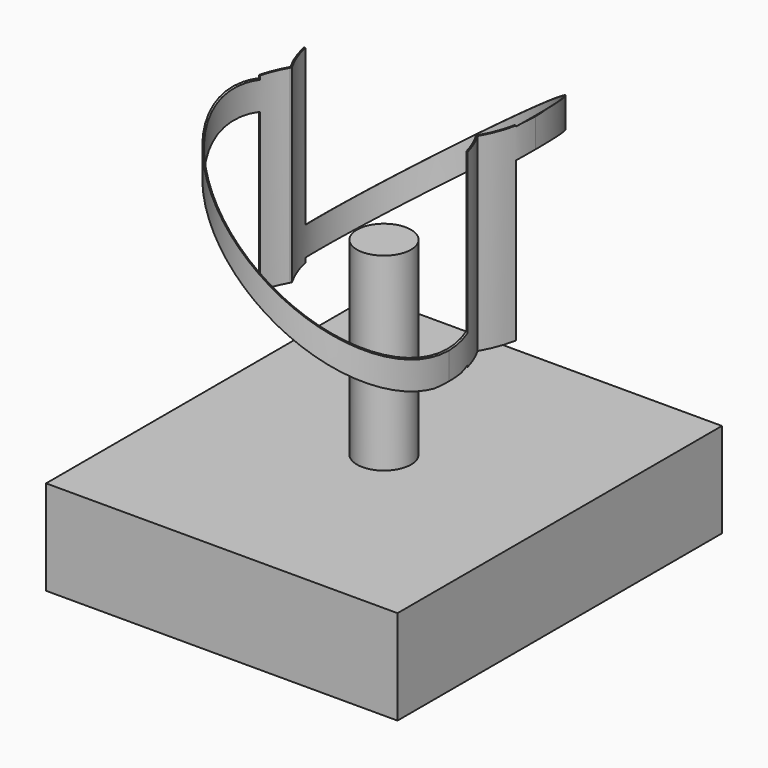
from build123d import *

# Parameters (mm, degrees)
F1_DEPTH = 35
F2_R     = 10
F3_DEPTH = 45
F5_DEPTH = 70
F7_DEPTH = 63
F9_DEPTH = 65.4


with BuildPart() as f1:
    # F0 (on Top) → F1 (new body)
    with BuildSketch(Plane.XY):
        Polygon((-147.9383396478, 75), (-147.9383396478, 0), (-147.9383396478, -75), (-17.9383396478, -75), (-17.9383396478, 0), (-17.9383396478, 75), align=None)
    extrude(amount=F1_DEPTH)

    # F2 (on face) → F3 (join)
    with BuildSketch(Plane.XY.offset(35)):
        with Locations((-82.9383396478, 0)):
            Circle(F2_R)
    extrude(amount=F3_DEPTH)

    # F2 (on face) → F5, piece 2 (join)
    with BuildSketch(Plane.XY.offset(35)):
        with Locations((-82.9383396478, 0)):
            Circle(F2_R)
    extrude(amount=F5_DEPTH)


with BuildPart() as f5:
    # F4 (on face) → F5 (new body)
    with BuildSketch(Plane.XY.offset(80)):
        with BuildLine():
            ThreePointArc((-48.5889857203, 0.496875), (-48.7315391647, 0.2479165476), (-48.8758969873, 0))
            ThreePointArc((-48.8758969873, 0), (-48.7315391647, -0.2479165476), (-48.5889857203, -0.496875))
            ThreePointArc((-48.5889857203, -0.496875), (-48.4422599851, -0.2489626377), (-48.2973234964, 0))
            ThreePointArc((-48.2973234964, 0), (-48.4422599851, 0.2489626377), (-48.5889857203, 0.496875))
        make_face()
        with BuildLine():
            ThreePointArc((-117.2876935753, -0.496875), (-117.1451401309, -0.2479165476), (-117.0007823083, 0))
            ThreePointArc((-117.0007823083, 0), (-117.1451401309, 0.2479165476), (-117.2876935753, 0.496875))
            ThreePointArc((-117.2876935753, 0.496875), (-117.4344193105, 0.2489626377), (-117.5793557992, 0))
            ThreePointArc((-117.5793557992, 0), (-117.4344193105, -0.2489626377), (-117.2876935753, -0.496875))
        make_face()
        with BuildLine():
            ThreePointArc((-43.4383396478, 20), (-44.7477028363, 9.9141058933), (-48.5889857203, 0.496875))
            ThreePointArc((-48.5889857203, 0.496875), (-48.4422599851, 0.2489626377), (-48.2973234964, 0))
            ThreePointArc((-48.2973234964, 0), (-44.3013065963, 9.6472381959), (-42.9383396478, 20))
            ThreePointArc((-42.9383396478, 20), (-93.2911014519, 58.6370330516), (-117.5793557992, 0))
            ThreePointArc((-117.5793557992, 0), (-117.4344193105, 0.2489626377), (-117.2876935753, 0.496875))
            ThreePointArc((-117.2876935753, 0.496875), (-93.0242337546, 58.1906368115), (-43.4383396478, 20))
        make_face()
        with BuildLine():
            ThreePointArc((-48.2973234964, 0), (-48.4422599851, -0.2489626377), (-48.5889857203, -0.496875))
            ThreePointArc((-48.5889857203, -0.496875), (-44.7477028363, -9.9141058933), (-43.4383396478, -20))
            ThreePointArc((-43.4383396478, -20), (-93.0242337546, -58.1906368115), (-117.2876935753, -0.496875))
            ThreePointArc((-117.2876935753, -0.496875), (-117.4344193105, -0.2489626377), (-117.5793557992, 0))
            ThreePointArc((-117.5793557992, 0), (-93.2911014519, -58.6370330516), (-42.9383396478, -20))
            ThreePointArc((-42.9383396478, -20), (-44.3013065963, -9.6472381959), (-48.2973234964, 0))
        make_face()
    extrude(amount=F5_DEPTH)

    # F6 (on face) → F7 (cut)
    with BuildSketch(Plane(origin=(0, 75, 0), x_dir=(-1, 0, 0), z_dir=(0, 1, 0))):
        Polygon((39.7482812405, 157.8890830278), (42.9177470505, 150.2823531628), (123.4222427011, 91.013289988), (145.2915817499, 160.4246497154), align=None)
        Polygon((125.323921442, 78.9693146944), (42.6008030772, 139.5061612129), (35.6279686093, 78.9693146944), (96.798710525, 78.9693146944), (115.498572588, 72.6303756237), align=None)
    extrude(amount=-F7_DEPTH, mode=Mode.SUBTRACT)

    # F8 (on face) → F9 (cut)
    with BuildSketch(Plane.XZ.offset(75)):
        Polygon((-33.7830297649, 154.05420959), (-123.1365576386, 150.1351892948), (-42.6008105278, 89.782372117), align=None)
        Polygon((-126.3355825414, 79.9848362803), (-42.6008105278, 79.3969780207), (-126.3355825414, 142.1471177791), align=None)
    extrude(amount=-F9_DEPTH, mode=Mode.SUBTRACT)


solid = Compound([f1.part, f5.part])
